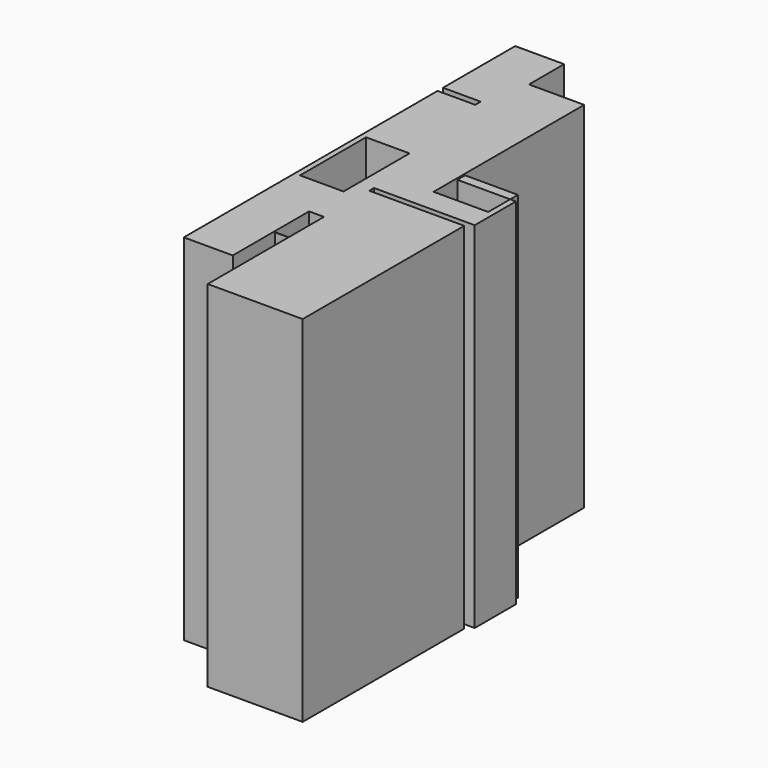
from build123d import *

# Parameters (mm, degrees)
F0_W     = 37.8432916477
F0_H     = 6.9169774652
F1_DEPTH = 254
F0_W_2   = 4.0263263509
F0_H_2   = 33.1595093012
F0_W_3   = 39.5476641133
F0_H_3   = 73.7544074655
F0_W_4   = 27.0056165755
F0_H_4   = 32.0053882897
F0_W_5   = 10.6641799212
F0_H_5   = 17.223265022
F0_W_6   = 34.8409274593
F0_W_7   = 3.8670822978
F0_H_6   = 1.6715824604
F0_H_7   = 30.8720460162
F0_W_8   = 0.7546879351
F0_H_8   = 30.3376843221
F0_W_9   = 9.626282379
F0_H_9   = 0.178348273


with BuildPart() as f1:
    # F0 (on Top) → F1 (new body)
    with BuildSketch(Plane.XY):
        with Locations((31.484158244, 79.1766680777)):
            Rectangle(F0_W, F0_H)
    extrude(amount=F1_DEPTH)


with BuildPart() as f1b:
    # F0 (on Top) → F1, piece 2 (new body)
    with BuildSketch(Plane.XY):
        Polygon((-28.2925348729, 222.3779112101), (-63.3508041501, 222.3779112101), (-63.3508041501, 190.9130513668), (-32.3188612238, 190.9130513668), (-28.2925348729, 190.9130513668), align=None)
        Polygon((-32.3188612238, 190.9130513668), (-63.3508041501, 190.9130513668), (-63.3508041501, 157.7535420656), (-36.3451875746, 157.7535420656), (-32.3188612238, 157.7535420656), align=None)
        with Locations((-30.3056980483, 174.3332967162)):
            Rectangle(F0_W_2, F0_H_2)
        with Locations((-8.5187028162, 174.3332967162)):
            Rectangle(F0_W_3, F0_H_2)
        Polygon((-28.2925348729, 83.9991346002), (-28.2925348729, 157.7535420656), (-32.3188612238, 157.7535420656), (-36.3451875746, 157.7535420656), (-36.3451875746, 152.8817266226), (-36.3451875746, 120.8763383329), (-36.3451875746, 83.9991346002), (-35.1700671017, 83.9991346002), (-30.1514100283, 83.9991346002), align=None)
        with Locations((-8.5187028162, 120.8763383329)):
            Rectangle(F0_W_3, F0_H_3)
        Polygon((11.2551292405, 83.9991346002), (-28.2925348729, 83.9991346002), (-28.2925348729, 82.3275521398), (-28.2925348729, 56.0619570315), (-17.6283549517, 56.0619570315), (11.2551292405, 56.0619570315), align=None)
        with Locations((-49.8479958624, 136.8790324777)):
            Rectangle(F0_W_4, F0_H_4)
        Polygon((-36.3451875746, 83.9991346002), (-36.3451875746, 120.8763383329), (-63.3508041501, 120.8763383329), (-63.3508041501, 83.9991346002), (-59.4837218523, 83.9991346002), align=None)
        Polygon((15.5648766086, 56.0619570315), (11.2551292405, 56.0619570315), (-17.6283549517, 56.0619570315), (-17.6283549517, 38.8386920094), (15.5648766086, 38.8386920094), align=None)
        with Locations((-22.9604449123, 47.4503245205)):
            Rectangle(F0_W_5, F0_H_5)
        with Locations((32.9853403382, 47.4503245205)):
            Rectangle(F0_W_6, F0_H_5)
        Polygon((-17.6283549517, 38.8386920094), (-28.2925348729, 38.8386920094), (-28.2925348729, 24.9053705484), (-17.6283549517, 24.9053705484), (-17.6283549517, 34.5843657851), align=None)
        with Locations((-61.4172630012, 83.16334337)):
            Rectangle(F0_W_7, F0_H_6)
        Polygon((50.4058040679, 75.7181793451), (50.4058040679, 56.0619570315), (50.4058040679, 38.8386920094), (54.5139685273, 38.8386920094), (54.5139685273, 75.7181793451), align=None)
        Polygon((-59.4837218523, 56.0619570315), (-59.4837218523, 82.3275521398), (-63.3508041501, 82.3275521398), (-63.3508041501, -74.2918476462), (-28.2925348729, -74.2918476462), (-28.2925348729, -37.5569090247), (-29.047222808, -37.5569090247), (-29.047222808, -7.2192247026), (-28.2925348729, -7.2192247026), (-28.2925348729, -5.9666754678), (-28.2925348729, 24.9053705484), (-48.5863350332, 24.9053705484), (-59.4837218523, 24.9053705484), align=None)
        with Locations((-22.9604449123, 9.4693475403)):
            Rectangle(F0_W_5, F0_H_7)
        Polygon((50.4058040679, 34.5843657851), (-17.6283549517, 34.5843657851), (-17.6283549517, 24.9053705484), (-17.6283549517, -5.9666754678), (-17.6283549517, -37.5569090247), (-17.6283549517, -37.7352572978), (-17.6283549517, -110.0548803806), (50.4058040679, -110.0548803806), align=None)
        with Locations((-28.6698788404, -22.3880668636)):
            Rectangle(F0_W_8, F0_H_8)
        with Locations((-22.4414961413, -37.6460831612)):
            Rectangle(F0_W_9, F0_H_9)
    extrude(amount=F1_DEPTH)


solid = Compound([f1.part, f1b.part])
